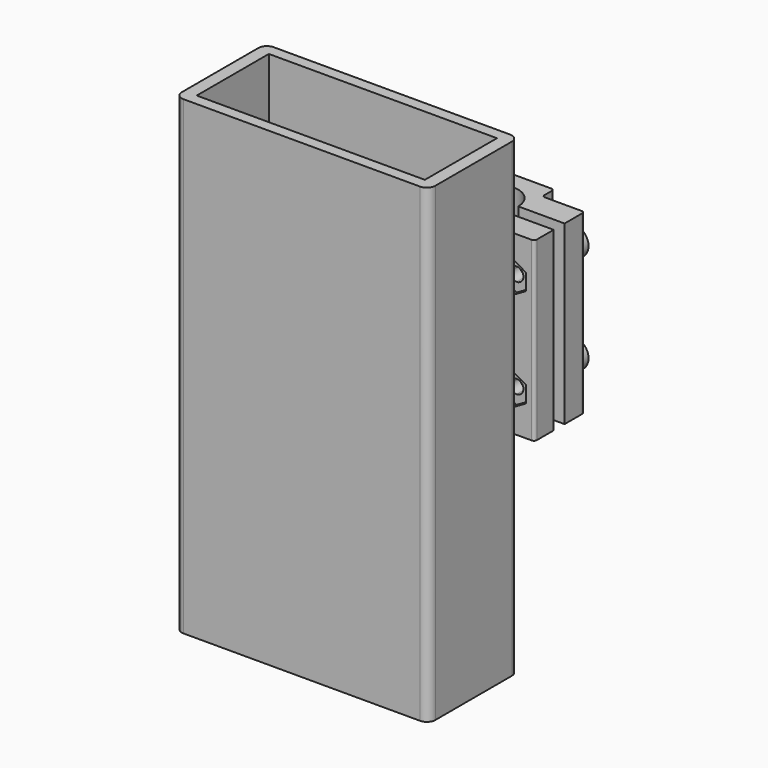
from build123d import *

# Parameters (mm, degrees)
F1_DEPTH  = 167
F0_W      = 6.2604716513
F0_H      = 5.1610916853
F2_DEPTH  = 55
F0_W_2    = 6.1
F0_H_2    = 5.2
F3_DEPTH  = 150
F6_DEPTH  = 85
F5_W      = 14
F5_H      = 52.1380715072
F5_W_2    = 14.3484344482
F5_W_3    = 7.8335499167
F5_W_4    = 7.4421485066
F7_DEPTH  = 85
F8_R      = 5
F8_R_2    = 2.425
F9_DEPTH  = 5.5
F10_DEPTH = 22
F12_DEPTH = 2
F13_DEPTH = 2
F14_R     = 4.979645
F14_R_2   = 2.425
F15_DEPTH = 2


# Not quite as in the source:
# - ends of sketch curves that miss each other by under 0.0002 mm in the source are joined
# - a feature names something its author has since deleted; it is built from what else it names


with BuildPart() as f1:
    # F0 (on Top) → F1 (new body)
    with BuildSketch(Plane.XY):
        with BuildLine():
            Line((-8.1248759852, 56.0848162174), (-24.5650857687, 56.0848162174))
            Line((-24.5650857687, 56.0848162174), (-24.5650857687, 48.5848162174))
            ThreePointArc((-24.5650857687, 48.5848162174), (-24.2721925499, 47.8777094362), (-23.5650857687, 47.5848162174))
            Line((-23.5650857687, 47.5848162174), (-10.5650857687, 47.5848162174))
            ThreePointArc((-10.5650857687, 47.5848162174), (-9.8579789875, 47.2919229986), (-9.5650857687, 46.5848162174))
            Line((-9.5650857687, 46.5848162174), (-9.5650857687, 32.5848162174))
            Line((-9.5650857687, 32.5848162174), (-3.1302364077, 32.5848162174))
            Line((-3.1302364077, 32.5848162174), (-3.1302364077, 37.7459079027))
            Line((-3.1302364077, 37.7459079027), (-6.7209850531, 37.7459079027))
            Line((-6.7209850531, 37.7459079027), (-6.7209850531, 43.8423007727))
            Line((-6.7209850531, 43.8423007727), (6.720983889, 43.8423007727))
            Line((6.720983889, 43.8423007727), (6.720983889, 37.7459079027))
            Line((6.720983889, 37.7459079027), (3.1302352436, 37.7459079027))
            Line((3.1302352436, 37.7459079027), (3.1302352436, 32.5848162174))
            Line((3.1302352436, 32.5848162174), (9.5650840085, 32.5848162174))
            Line((9.5650840085, 32.5848162174), (9.5650834125, 46.5848162174))
            ThreePointArc((9.5650834125, 46.5848162174), (9.8579766313, 47.2919229986), (10.5650834125, 47.5848162174))
            Line((10.5650834125, 47.5848162174), (23.5650834125, 47.5848162174))
            ThreePointArc((23.5650834125, 47.5848162174), (24.2721901936, 47.8777094362), (24.5650834125, 48.5848162174))
            Line((24.5650834125, 48.5848162174), (24.5650834125, 56.0848162174))
            Line((24.5650834125, 56.0848162174), (8.1248747931, 56.0848162174))
            ThreePointArc((8.1248747931, 56.0848162174), (5.7293103589, 50.3686850456), (-5.96e-07, 48.0048152283))
            ThreePointArc((-5.96e-07, 48.0048152283), (-5.729311551, 50.3686850456), (-8.1248759852, 56.0848162174))
        make_face()
    extrude(amount=F1_DEPTH)

    # F0 (on Top) → F2 (join)
    with BuildSketch(Plane.XY):
        Polygon((-6.7209850531, 37.7459079027), (-3.1302364077, 37.7459079027), (3.1302352436, 37.7459079027), (6.720983889, 37.7459079027), (6.720983889, 43.8423007727), (-6.7209850531, 43.8423007727), align=None)
        with Locations((-5.821e-07, 35.1653620601)):
            Rectangle(F0_W, F0_H)
    extrude(amount=F2_DEPTH)


with BuildPart() as f1b:
    # F0 (on Top) → F1, piece 2 (new body)
    with BuildSketch(Plane.XY):
        with BuildLine():
            Line((41.9999994179, 15), (10.5650840085, 15))
            Line((10.5650840085, 15), (-5.821e-07, 15))
            Line((-5.821e-07, 15), (-10.565086104, 15))
            Line((-10.565086104, 15), (-42.0000005821, 15))
            ThreePointArc((-42.0000005821, 15), (-44.1213209256, 14.1213203436), (-45.0000005821, 12))
            Line((-45.0000005821, 12), (-45.0000005821, -22.0000006706))
            ThreePointArc((-45.0000005821, -22.0000006706), (-44.1213209256, -24.1213210141), (-42.0000005821, -25.0000006706))
            Line((-42.0000005821, -25.0000006706), (41.9999994179, -25.0000006706))
            ThreePointArc((41.9999994179, -25.0000006706), (44.1213197615, -24.1213210141), (44.9999994179, -22.0000006706))
            Line((44.9999994179, -22.0000006706), (44.9999994179, 12))
            ThreePointArc((44.9999994179, 12), (44.1213197615, 14.1213203436), (41.9999994179, 15))
        make_face()
        Polygon((40.4999994179, 10.9999996647), (40.4999994179, -21.0000003353), (-40.5000005821, -21.0000003353), (-40.5000005821, 10.9999996647), (0, 10.9999996647), align=None, mode=Mode.SUBTRACT)
    extrude(amount=F1_DEPTH)

    # F0 (on Top) → F3 (join)
    with BuildSketch(Plane.XY):
        with BuildLine():
            ThreePointArc((10.5650840085, 15), (9.8579772273, 15.2928932188), (9.5650840085, 16))
            Line((9.5650840085, 16), (9.5650840085, 18.8283249736))
            Line((9.5650840085, 18.8283249736), (3.0499994179, 18.8283249736))
            Line((3.0499994179, 18.8283249736), (-3.0500005821, 18.8283249736))
            Line((-3.0500005821, 18.8283249736), (-9.565086104, 18.8283249736))
            Line((-9.565086104, 18.8283249736), (-9.565086104, 16))
            ThreePointArc((-9.565086104, 16), (-9.8579793228, 15.2928932188), (-10.565086104, 15))
            Line((-10.565086104, 15), (-5.821e-07, 15))
            Line((-5.821e-07, 15), (10.5650840085, 15))
        make_face()
        with Locations((-5.821e-07, 21.4283249736)):
            Rectangle(F0_W_2, F0_H_2)
        Polygon((-3.0500005821, 24.0283246636), (3.0499994179, 24.0283246636), (6.6499994179, 24.0283246636), (6.6499994179, 30.0283246636), (-6.6500005821, 30.0283246636), (-6.6500005821, 24.0283246636), align=None)
    extrude(amount=F3_DEPTH)

    # F4 (on face) → F6 (cut)
    with BuildSketch(Plane(origin=(-24.5650857687, 0, 0), x_dir=(0, -1, 0), z_dir=(-1, 0, 0))):
        with BuildLine():
            Line((-32.5848162174, 0), (-14.9999996647, 0))
            Line((-14.9999996647, 0), (-14.9999996647, 48))
            ThreePointArc((-14.9999996647, 48), (-17.0502521964, 52.9497474683), (-21.9999996647, 55))
            Line((-21.9999996647, 55), (-32.5848162174, 55))
            Line((-32.5848162174, 55), (-32.5848162174, 0))
        make_face()
        with BuildLine():
            Line((-14.9999996647, 119.0000034571), (-14.9999996647, 167.0000034571))
            Line((-14.9999996647, 167.0000034571), (-32.5848162174, 167.0000034571))
            Line((-32.5848162174, 167.0000034571), (-32.5848162174, 112.0000034571))
            Line((-32.5848162174, 112.0000034571), (-21.9999996647, 112.0000034571))
            ThreePointArc((-21.9999996647, 112.0000034571), (-17.0502521964, 114.0502559888), (-14.9999996647, 119.0000034571))
        make_face()
    extrude(amount=-F6_DEPTH, mode=Mode.SUBTRACT)

    # F0 (on Top) → F13 (join)
    with BuildSketch(Plane.XY):
        Polygon((-40.5000005821, -21.0000003353), (40.4999994179, -21.0000003353), (40.4999994179, 10.9999996647), (0, 10.9999996647), (-40.5000005821, 10.9999996647), align=None)
        with BuildLine():
            ThreePointArc((-21.650703999, 8.016124128), (-15.9938497495, 5.6729783775), (-13.650703999, 0.016124128))
            ThreePointArc((-13.650703999, 0.016124128), (-27.3075582485, -5.6407301215), (-21.650703999, 8.016124128))
        make_face(mode=Mode.SUBTRACT)
        Polygon((-5.8, 2.4249994893), (0, 2.4249994893), (5.8, 2.4249994893), (5.8, -9.2250005107), (0, -9.2250005107), (-5.8, -9.2250005107), (-5.8, -0.8999999845), align=None, mode=Mode.SUBTRACT)
        with BuildLine():
            ThreePointArc((21.6507028348, 8.016124128), (27.3075570843, 5.6729783775), (29.6507028348, 0.016124128))
            ThreePointArc((29.6507028348, 0.016124128), (15.9938485853, -5.6407301215), (21.6507028348, 8.016124128))
        make_face(mode=Mode.SUBTRACT)
    extrude(amount=F13_DEPTH)


with BuildPart() as f1c:
    # F0 (on Top) → F1, piece 3 (new body)
    with BuildSketch(Plane.XY):
        with BuildLine():
            Line((19.2612114083, 60.9332506657), (24.5650835615, 60.9332506657))
            Line((24.5650835615, 60.9332506657), (24.5650835615, 68.4332506657))
            Line((24.5650835615, 68.4332506657), (24.5650835615, 68.7668005824))
            ThreePointArc((24.5650835615, 68.7668005824), (24.2721903427, 69.4739073636), (23.5650835615, 69.7668005824))
            Line((23.5650835615, 69.7668005824), (10.5650840085, 69.7668005824))
            ThreePointArc((10.5650840085, 69.7668005824), (9.8579772273, 70.0596938012), (9.5650840085, 70.7668005824))
            Line((9.5650840085, 70.7668005824), (9.5650840085, 74.024710536))
            ThreePointArc((9.5650840085, 74.024710536), (9.2721907897, 74.7318173172), (8.5650840085, 75.024710536))
            Line((8.5650840085, 75.024710536), (-8.5650851727, 75.024710536))
            ThreePointArc((-8.5650851727, 75.024710536), (-9.2721919538, 74.7318173172), (-9.5650851727, 74.024710536))
            Line((-9.5650851727, 74.024710536), (-9.5650851727, 70.7668005824))
            ThreePointArc((-9.5650851727, 70.7668005824), (-9.8579783915, 70.0596938012), (-10.5650851727, 69.7668005824))
            Line((-10.5650851727, 69.7668005824), (-23.5650856197, 69.7668005824))
            ThreePointArc((-23.5650856197, 69.7668005824), (-24.2721924009, 69.4739073636), (-24.5650856197, 68.7668005824))
            Line((-24.5650856197, 68.7668005824), (-24.5650856197, 68.4332506657))
            Line((-24.5650856197, 68.4332506657), (-24.5650856197, 60.9332506657))
            Line((-24.5650856197, 60.9332506657), (-19.2612134665, 60.9332506657))
            Line((-19.2612134665, 60.9332506657), (-8.1248758362, 60.9332506657))
            ThreePointArc((-8.1248758362, 60.9332506657), (-5.7293114548, 66.6493817849), (-5.96e-07, 69.0132516548))
            ThreePointArc((-5.96e-07, 69.0132516548), (5.7293104551, 66.64938189), (8.1248749421, 60.9332506657))
            Line((8.1248749421, 60.9332506657), (19.2612114083, 60.9332506657))
        make_face()
    extrude(amount=F1_DEPTH)


with BuildPart() as f7_tool:
    # F5 (on face) → F7 (new body)
    with BuildSketch(Plane(origin=(-24.5650856197, 0, 0), x_dir=(0, -1, 0), z_dir=(-1, 0, 0))):
        with Locations((-39.5848162174, 140.9309642464)):
            Rectangle(F5_W, F5_H)
        with Locations((-39.5848162174, 26.0690357536)):
            Rectangle(F5_W, F5_H)
        with Locations((-53.7590334415, 140.9309642464)):
            Rectangle(F5_W_2, F5_H)
        with Locations((-64.850025624, 140.9309642464)):
            Rectangle(F5_W_3, F5_H)
        with Locations((-72.4878748357, 140.9309642464)):
            Rectangle(F5_W_4, F5_H)
        with Locations((-53.7590334415, 26.0690357536)):
            Rectangle(F5_W_2, F5_H)
        with Locations((-64.850025624, 26.0690357536)):
            Rectangle(F5_W_3, F5_H)
        with Locations((-72.4878748357, 26.0690357536)):
            Rectangle(F5_W_4, F5_H)
    extrude(amount=-F7_DEPTH)


with BuildPart() as f1_1:
    add(f1.part)

    # F7: cut by f7_tool
    add(f7_tool.part, mode=Mode.SUBTRACT)


with BuildPart() as f1c_1:
    add(f1c.part)

    # F7: cut by f7_tool
    add(f7_tool.part, mode=Mode.SUBTRACT)

    # F8 (on face) → F9 (join)
    with BuildSketch(Plane(origin=(0, 69.7668005824, 0), x_dir=(-1, 0, 0), z_dir=(0, 1, 0))):
        with BuildLine():
            Line((-16.610749317, 103.4829019785), (-16.610749317, 106.0579019785))
            ThreePointArc((-16.610749317, 106.0579019785), (-21.610749317, 101.0579019785), (-16.610749317, 96.0579019785))
            Line((-16.610749317, 96.0579019785), (-16.610749317, 98.6329019785))
            ThreePointArc((-16.610749317, 98.6329019785), (-19.035749317, 101.0579019785), (-16.610749317, 103.4829019785))
        make_face()
        with BuildLine():
            ThreePointArc((-11.610749317, 101.0579019785), (-13.075215411, 104.5934358844), (-16.610749317, 106.0579019785))
            Line((-16.610749317, 106.0579019785), (-16.610749317, 103.4829019785))
            ThreePointArc((-16.610749317, 103.4829019785), (-14.8960153726, 102.7726359229), (-14.185749317, 101.0579019785))
            ThreePointArc((-14.185749317, 101.0579019785), (-14.8960153726, 99.3431680341), (-16.610749317, 98.6329019785))
            Line((-16.610749317, 98.6329019785), (-16.610749317, 96.0579019785))
            ThreePointArc((-16.610749317, 96.0579019785), (-13.075215411, 97.5223680726), (-11.610749317, 101.0579019785))
        make_face()
        with BuildLine():
            Line((-16.610749317, 68.3670980215), (-16.610749317, 70.9420980215))
            ThreePointArc((-16.610749317, 70.9420980215), (-21.610749317, 65.9420980215), (-16.610749317, 60.9420980215))
            Line((-16.610749317, 60.9420980215), (-16.610749317, 63.5170980215))
            ThreePointArc((-16.610749317, 63.5170980215), (-19.035749317, 65.9420980215), (-16.610749317, 68.3670980215))
        make_face()
        with BuildLine():
            ThreePointArc((-11.610749317, 65.9420980215), (-13.075215411, 69.4776319274), (-16.610749317, 70.9420980215))
            Line((-16.610749317, 70.9420980215), (-16.610749317, 68.3670980215))
            ThreePointArc((-16.610749317, 68.3670980215), (-14.8960153726, 67.6568319659), (-14.185749317, 65.9420980215))
            ThreePointArc((-14.185749317, 65.9420980215), (-14.8960153726, 64.2273640771), (-16.610749317, 63.5170980215))
            Line((-16.610749317, 63.5170980215), (-16.610749317, 60.9420980215))
            ThreePointArc((-16.610749317, 60.9420980215), (-13.075215411, 62.4065641156), (-11.610749317, 65.9420980215))
        make_face()
        with Locations((16.610749317, 101.0579019785)):
            Circle(F8_R)
        with Locations((16.610749317, 101.0579019785)):
            Circle(F8_R_2, mode=Mode.SUBTRACT)
        with Locations((16.610749317, 65.9420980215)):
            Circle(F8_R)
        with Locations((16.610749317, 65.9420980215)):
            Circle(F8_R_2, mode=Mode.SUBTRACT)
    extrude(amount=F9_DEPTH)


with BuildPart() as f10_tool:
    # F8 (on face) → F10 (new body)
    with BuildSketch(Plane(origin=(0, 69.7668005824, 0), x_dir=(-1, 0, 0), z_dir=(0, 1, 0))):
        with BuildLine():
            Line((-16.610749317, 98.6329019785), (-16.610749317, 103.4829019785))
            ThreePointArc((-16.610749317, 103.4829019785), (-19.035749317, 101.0579019785), (-16.610749317, 98.6329019785))
        make_face()
        with BuildLine():
            ThreePointArc((-14.185749317, 101.0579019785), (-14.8960153726, 102.7726359229), (-16.610749317, 103.4829019785))
            Line((-16.610749317, 103.4829019785), (-16.610749317, 98.6329019785))
            ThreePointArc((-16.610749317, 98.6329019785), (-14.8960153726, 99.3431680341), (-14.185749317, 101.0579019785))
        make_face()
        with Locations((16.610749317, 101.0579019785)):
            Circle(F8_R_2)
        with Locations((16.610749317, 65.9420980215)):
            Circle(F8_R_2)
        with BuildLine():
            Line((-16.610749317, 63.5170980215), (-16.610749317, 68.3670980215))
            ThreePointArc((-16.610749317, 68.3670980215), (-19.035749317, 65.9420980215), (-16.610749317, 63.5170980215))
        make_face()
        with BuildLine():
            ThreePointArc((-14.185749317, 65.9420980215), (-14.8960153726, 67.6568319659), (-16.610749317, 68.3670980215))
            Line((-16.610749317, 68.3670980215), (-16.610749317, 63.5170980215))
            ThreePointArc((-16.610749317, 63.5170980215), (-14.8960153726, 64.2273640771), (-14.185749317, 65.9420980215))
        make_face()
    extrude(amount=-F10_DEPTH)


with BuildPart() as f1_2:
    add(f1_1.part)

    # F10: cut by f10_tool
    add(f10_tool.part, mode=Mode.SUBTRACT)

    # F11 (on face) → F12 (cut)
    with BuildSketch(Plane.XZ.offset(-47.5848162174)):
        Polygon((-11.6311032452, 98.1829019785), (-11.6311032452, 103.9329019785), (-16.610749317, 106.8079019785), (-21.5903953887, 103.9329019785), (-21.5903953887, 98.1829019785), (-16.610749317, 95.3079019785), align=None)
        Polygon((-11.6311032452, 63.0670980215), (-11.6311032452, 68.8170980215), (-16.610749317, 71.6920980215), (-21.5903953887, 68.8170980215), (-21.5903953887, 63.0670980215), (-16.610749317, 60.1920980215), align=None)
        Polygon((11.6311032452, 103.9329019785), (11.6311032452, 98.1829019785), (16.610749317, 95.3079019785), (21.5903953887, 98.1829019785), (21.5903953887, 103.9329019785), (16.610749317, 106.8079019785), align=None)
        Polygon((11.6311032452, 68.8170980215), (11.6311032452, 63.0670980215), (16.610749317, 60.1920980215), (21.5903953887, 63.0670980215), (21.5903953887, 68.8170980215), (16.610749317, 71.6920980215), align=None)
    extrude(amount=-F12_DEPTH, mode=Mode.SUBTRACT)

    # F14 (on face) → F15 (cut)
    with BuildSketch(Plane(origin=(0, 56.0848162174, 0), x_dir=(-1, 0, 0), z_dir=(0, 1, 0))):
        with Locations((16.610749317, 101.0579019785)):
            Circle(F14_R)
        with Locations((16.610749317, 101.0579019785)):
            Circle(F14_R_2, mode=Mode.SUBTRACT)
        with Locations((16.610749317, 65.9420980215)):
            Circle(F14_R)
        with Locations((16.610749317, 65.9420980215)):
            Circle(F14_R_2, mode=Mode.SUBTRACT)
        with Locations((-16.610749317, 65.9420980215)):
            Circle(F14_R)
        with Locations((-16.610749317, 101.0579019785)):
            Circle(F14_R)
    extrude(amount=-F15_DEPTH, mode=Mode.SUBTRACT)


with BuildPart() as f1c_2:
    add(f1c_1.part)

    # F10: cut by f10_tool
    add(f10_tool.part, mode=Mode.SUBTRACT)


solid = Compound([f1b.part, f1_2.part, f1c_2.part])
